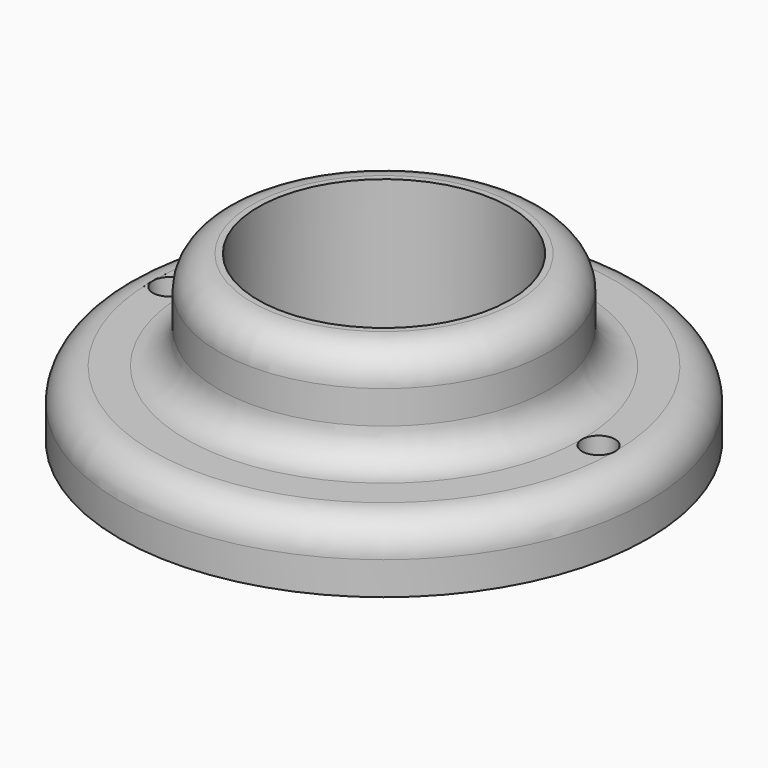
from build123d import *

# Parameters (mm, degrees)
F0_R     = 25
F0_R_2   = 19.066290696
F1_DEPTH = 25
F0_R_3   = 40
F0_R_4   = 2.5
F2_DEPTH = 10
F3_R     = 4.99999
F4_R     = 4.99999


# Not quite as in the source:
# - a fillet or chamfer is up to 0.001 mm smaller than in the source, because OpenCascade refuses the exact size


with BuildPart() as f1:
    # F0 (on Top) → F1 (new body)
    with BuildSketch(Plane.XY):
        Circle(F0_R)
        Circle(F0_R_2, mode=Mode.SUBTRACT)
    extrude(amount=F1_DEPTH)

    # F0 (on Top) → F2 (join)
    with BuildSketch(Plane.XY):
        Circle(F0_R_3)
        with Locations((-32.5, 0)):
            Circle(F0_R_4, mode=Mode.SUBTRACT)
        Circle(F0_R, mode=Mode.SUBTRACT)
        with Locations((32.5, 0)):
            Circle(F0_R_4, mode=Mode.SUBTRACT)
    extrude(amount=F2_DEPTH)

    # F3 (radius 5 in the source; OpenCascade refuses exactly that, so slightly less here)
    f3_edges = [f1.edges().sort_by_distance(p)[0] for p in [
        (-40, 0, 10),
        (-25, 0, 25),
    ]]
    fillet(f3_edges, radius=F3_R)

    # F4 (radius 5 in the source; OpenCascade refuses exactly that, so slightly less here)
    f4_edges = [f1.edges().sort_by_distance(p)[0] for p in [
        (25, 0, 15.000005),
        (-25, 0, 20.00001),
        (-25, 0, 10),
    ]]
    fillet(f4_edges, radius=F4_R)


solid = f1.part
